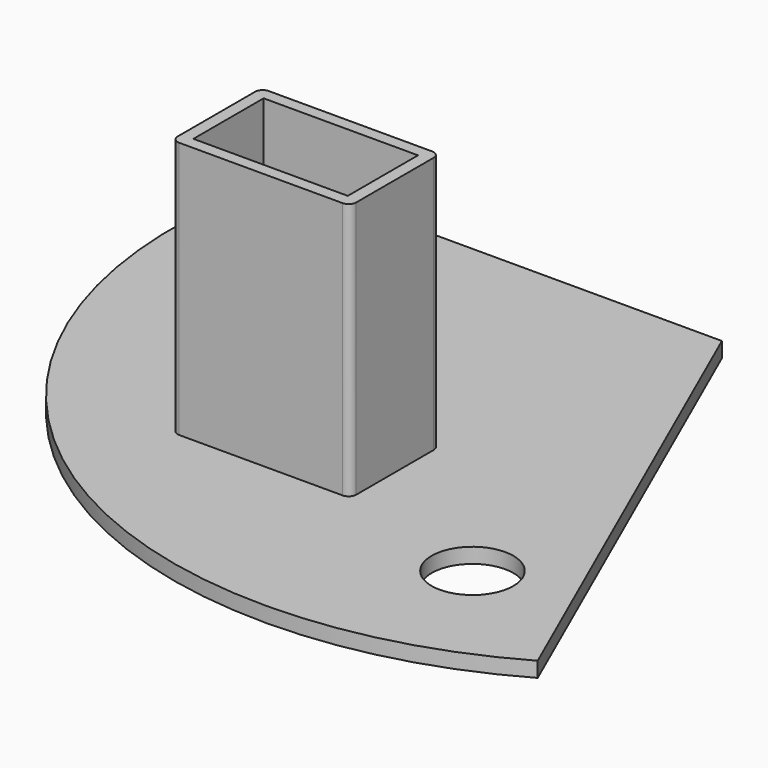
from build123d import *

# Parameters (mm, degrees)
F0_R     = 2.7
F1_DEPTH = 1
F2_DEPTH = 18


# Not quite as in the source:
# - a feature names something its author has since deleted; it is built from what else it names


with BuildPart() as f1:
    # F0 (on Top) → F1 (new body)
    with BuildSketch(Plane.XY):
        with BuildLine():
            Line((0, 7.8000635883), (-28.9682413691, 7.8000635883))
            ThreePointArc((-28.9682413691, 7.8000635883), (-18.3237536434, -23.7537376515), (14.8986014601, -26.039041352))
            Line((14.8986014601, -26.039041352), (0, 7.8000635883))
        make_face()
        with BuildLine():
            ThreePointArc((-9.6558443136, -17.9), (-21.5, -14.2), (-9.6558443136, -10.5))
            Line((-9.6558443136, -10.5), (-4.5, -10.5))
            ThreePointArc((-4.5, -10.5), (-4.1464466094, -10.6464466094), (-4, -11))
            Line((-4, -11), (-4, -17.4))
            ThreePointArc((-4, -17.4), (-4.1464466094, -17.7535533906), (-4.5, -17.9))
            Line((-4.5, -17.9), (-9.6558443136, -17.9))
        make_face(mode=Mode.SUBTRACT)
        with Locations((6, -20.3)):
            Circle(F0_R, mode=Mode.SUBTRACT)
        with Locations((-21, 2.5)):
            Circle(F0_R, mode=Mode.SUBTRACT)
        with BuildLine():
            Line((-15.3, -10.5), (-9.6558443136, -10.5))
            ThreePointArc((-9.6558443136, -10.5), (-21.5, -14.2), (-9.6558443136, -17.9))
            Line((-9.6558443136, -17.9), (-15.3, -17.9))
            ThreePointArc((-15.3, -17.9), (-15.6535533906, -17.7535533906), (-15.8, -17.4))
            Line((-15.8, -17.4), (-15.8, -11))
            ThreePointArc((-15.8, -11), (-15.6535533906, -10.6464466094), (-15.3, -10.5))
        make_face()
        with BuildLine():
            Line((-15, -11.3), (-9.1827841711, -11.3))
            ThreePointArc((-9.1827841711, -11.3), (-9.4049974508, -10.8915341207), (-9.6558443136, -10.5))
            Line((-9.6558443136, -10.5), (-15.3, -10.5))
            ThreePointArc((-15.3, -10.5), (-15.6535533906, -10.6464466094), (-15.8, -11))
            Line((-15.8, -11), (-15.8, -17.4))
            ThreePointArc((-15.8, -17.4), (-15.6535533906, -17.7535533906), (-15.3, -17.9))
            Line((-15.3, -17.9), (-9.6558443136, -17.9))
            ThreePointArc((-9.6558443136, -17.9), (-9.4049974508, -17.5084658793), (-9.1827841711, -17.1))
            Line((-9.1827841711, -17.1), (-15, -17.1))
            Line((-15, -17.1), (-15, -11.3))
        make_face()
        with BuildLine():
            ThreePointArc((-9.6558443136, -10.5), (-9.4049974508, -10.8915341207), (-9.1827841711, -11.3))
            Line((-9.1827841711, -11.3), (-4.8, -11.3))
            Line((-4.8, -11.3), (-4.8, -17.1))
            Line((-4.8, -17.1), (-9.1827841711, -17.1))
            ThreePointArc((-9.1827841711, -17.1), (-9.4049974508, -17.5084658793), (-9.6558443136, -17.9))
            Line((-9.6558443136, -17.9), (-4.5, -17.9))
            ThreePointArc((-4.5, -17.9), (-4.1464466094, -17.7535533906), (-4, -17.4))
            Line((-4, -17.4), (-4, -11))
            ThreePointArc((-4, -11), (-4.1464466094, -10.6464466094), (-4.5, -10.5))
            Line((-4.5, -10.5), (-9.6558443136, -10.5))
        make_face()
        with BuildLine():
            ThreePointArc((-9.1827841711, -11.3), (-8.6729982263, -12.7103528753), (-8.5, -14.2))
            ThreePointArc((-8.5, -14.2), (-8.6729982263, -15.6896471247), (-9.1827841711, -17.1))
            Line((-9.1827841711, -17.1), (-4.8, -17.1))
            Line((-4.8, -17.1), (-4.8, -11.3))
            Line((-4.8, -11.3), (-9.1827841711, -11.3))
        make_face()
    extrude(amount=F1_DEPTH)

    # F0 (on Top) → F2 (join)
    with BuildSketch(Plane.XY):
        with BuildLine():
            Line((-15, -11.3), (-9.1827841711, -11.3))
            ThreePointArc((-9.1827841711, -11.3), (-9.4049974508, -10.8915341207), (-9.6558443136, -10.5))
            Line((-9.6558443136, -10.5), (-15.3, -10.5))
            ThreePointArc((-15.3, -10.5), (-15.6535533906, -10.6464466094), (-15.8, -11))
            Line((-15.8, -11), (-15.8, -17.4))
            ThreePointArc((-15.8, -17.4), (-15.6535533906, -17.7535533906), (-15.3, -17.9))
            Line((-15.3, -17.9), (-9.6558443136, -17.9))
            ThreePointArc((-9.6558443136, -17.9), (-9.4049974508, -17.5084658793), (-9.1827841711, -17.1))
            Line((-9.1827841711, -17.1), (-15, -17.1))
            Line((-15, -17.1), (-15, -11.3))
        make_face()
        with BuildLine():
            ThreePointArc((-9.6558443136, -10.5), (-9.4049974508, -10.8915341207), (-9.1827841711, -11.3))
            Line((-9.1827841711, -11.3), (-4.8, -11.3))
            Line((-4.8, -11.3), (-4.8, -17.1))
            Line((-4.8, -17.1), (-9.1827841711, -17.1))
            ThreePointArc((-9.1827841711, -17.1), (-9.4049974508, -17.5084658793), (-9.6558443136, -17.9))
            Line((-9.6558443136, -17.9), (-4.5, -17.9))
            ThreePointArc((-4.5, -17.9), (-4.1464466094, -17.7535533906), (-4, -17.4))
            Line((-4, -17.4), (-4, -11))
            ThreePointArc((-4, -11), (-4.1464466094, -10.6464466094), (-4.5, -10.5))
            Line((-4.5, -10.5), (-9.6558443136, -10.5))
        make_face()
    extrude(amount=F2_DEPTH)


solid = f1.part
